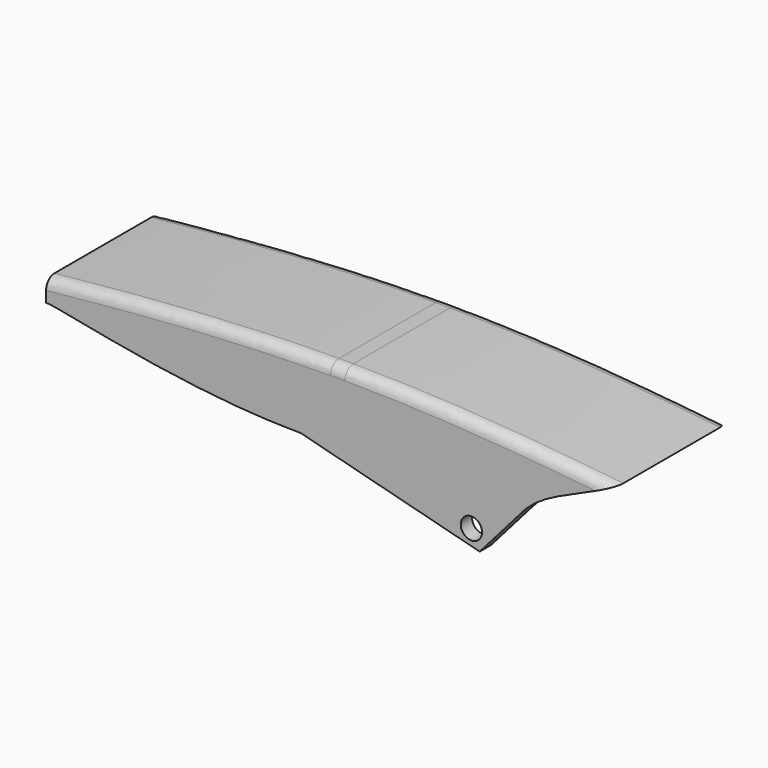
from build123d import *

# Parameters (mm, degrees)
F1_DEPTH    = 200
F2_R        = 15
F4_DEPTH    = 15
F5_W        = 259.7017054144
F5_H        = 160
F6_DEPTH    = 50
F7_T1_DEPTH = 160
F8_R        = 15
F9_DEPTH    = 300


# Not quite as in the source:
# - a fillet or chamfer that OpenCascade refuses, or shapes differently, is made with other operations: its cross-section is extruded or revolved along the edge and cut away or added


with BuildPart() as f1:
    # F0 (on Front) → F1 (new body)
    with BuildSketch(Plane.XZ):
        with BuildLine():
            add(Edge.make_bspline(
                [(20.2008041868, 100), (146.0822657859, 99.5052919304), (265.431836351, 89.8162356005), (400, 75.4941478372)],
                knots=[0.5253173238, 0.5253173238, 0.5253173238, 0.5253173238, 1, 1, 1, 1], degree=3))
            Line((20.2008041868, 100), (0, 100))
            add(Edge.make_bspline(
                [(-400, 75.4941478372), (-275.3232982272, 88.4775108691), (-133.3944766528, 99.4743507493), (0, 100)],
                knots=[0, 0, 0, 0, 0.5, 0.5, 0.5, 0.5], degree=3))
            Line((-400, 75.4941478372), (-400, 44.4300249219))
            add(Edge.make_bspline(
                [(-41.6261814535, 0), (-214.6242707968, 0), (-393.6260249555, 49.33328574), (-400, 44.4300249219)],
                knots=[0, 0, 0, 0, 0.9473133281, 0.9473133281, 0.9473133281, 0.9473133281], degree=3))
            Line((-41.6261814535, 0), (209.8438292742, -64.8676306009))
            Line((209.8438292742, -64.8676306009), (266.6716873646, 0))
            add(Edge.make_bspline(
                [(400, 75.4941478372), (313.5865926743, 36.6108752787), (291.246175766, 29.9087464809), (266.6716873646, 0)],
                knots=[0, 0, 0, 0, 153.2181624608, 153.2181624608, 153.2181624608, 153.2181624608], degree=3))
        make_face()
    extrude(amount=F1_DEPTH)

    # F2
    f2_edges = [f1.edges().sort_by_distance(p)[0] for p in [
        (-200.289149, -200, 92.61289),
        (210.407204, -200, 92.68637),
        (-200.289149, 0, 92.61289),
        (10.100402, -200, 100),
        (10.100402, 0, 100),
        (210.407204, 0, 92.68637),
    ]]
    fillet(f2_edges, radius=F2_R)

    # F3 (on face) → F4 (cut, symmetric)
    with BuildSketch(Plane(origin=(150.8768626718, 0, -132.1770020211), x_dir=(0, 1, 0), z_dir=(0.7521818814, 0, -0.6589555503))):
        with BuildLine():
            Line((-180, 226.1682897806), (-180, 89.4854995586))
            Line((-180, 89.4854995586), (-20, 89.4854995586))
            Line((-20, 89.4854995586), (-20, 226.1682897806))
            add(Edge.make_bspline(
                [(-180, 226.1682897806), (-153.3333333333, 247.7404251695), (-100, 290.8846959472), (-46.6666666667, 247.7404251695), (-20, 226.1682897806)],
                knots=[0, 0, 0, 0, 0.5, 1, 1, 1, 1], degree=3))
        make_face()
    extrude(amount=F4_DEPTH, both=True, mode=Mode.SUBTRACT)

    # F5 (on face) → F6 (cut)
    with BuildSketch(Plane(origin=(-2.5970065182, 0, -10.0677217734), x_dir=(0.9683032706, 0, -0.2497774533), z_dir=(-0.2497774533, 0, -0.9683032706))):
        with Locations((89.5440850641, 100)):
            Rectangle(F5_W, F5_H)
    extrude(amount=-F6_DEPTH, mode=Mode.SUBTRACT)

    # F7: fillet of radius 15 on 1 edges, made by hand

    # F7_s2 → F7_t1 (cut)
    with BuildSketch(Plane.XZ.offset(20)):
        with BuildLine():
            ThreePointArc((236.54494855, -11.6256507443), (230.0859706945, -15.9445365763), (222.3327019401, -16.452467072))
            Line((222.3327019401, -16.452467072), (218.1662168076, -32.6045301468))
            Line((218.1662168076, -32.6045301468), (236.54494855, -11.6256507443))
        make_face()
    extrude(amount=F7_T1_DEPTH, mode=Mode.SUBTRACT)

    # F8 (on face) → F9 (cut)
    with BuildSketch(Plane.XZ.offset(200)):
        with Locations((198.1902569532, -39.8889631033)):
            Circle(F8_R)
    extrude(amount=-F9_DEPTH, mode=Mode.SUBTRACT)


solid = f1.part
